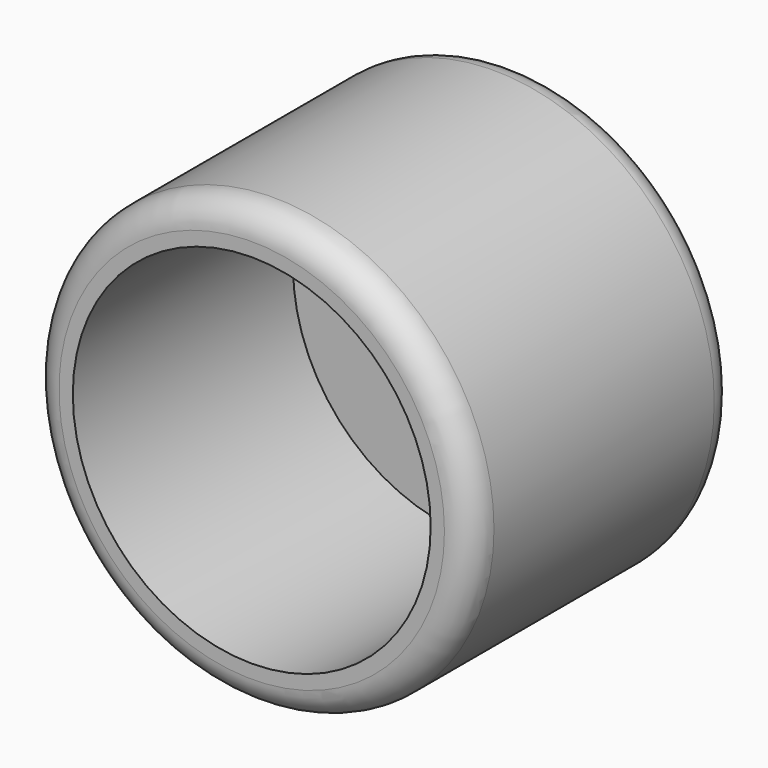
from build123d import *

# Parameters (mm, degrees)
F0_R     = 8
F0_R_2   = 6.5
F1_DEPTH = 12
F2_R     = 1
F3_R     = 7
F3_R_2   = 6.5
F4_DEPTH = 2


with BuildPart() as f1:
    # F0 (on Front) → F1 (new body)
    with BuildSketch(Plane.XZ):
        Circle(F0_R)
        Circle(F0_R_2, mode=Mode.SUBTRACT)
    extrude(amount=F1_DEPTH)

    # F2
    f2_edges = [f1.edges().sort_by_distance(p)[0] for p in [
        (-8, -12, 0),
        (-8, 0, 0),
    ]]
    fillet(f2_edges, radius=F2_R)

    # F3 (on face) → F4 (join)
    with BuildSketch(Plane(origin=(0, 0, 0), x_dir=(-1, 0, 0), z_dir=(0, 1, 0))):
        Circle(F3_R)
        Circle(F3_R_2, mode=Mode.SUBTRACT)
        Circle(F3_R_2)
    extrude(amount=-F4_DEPTH)


solid = f1.part
